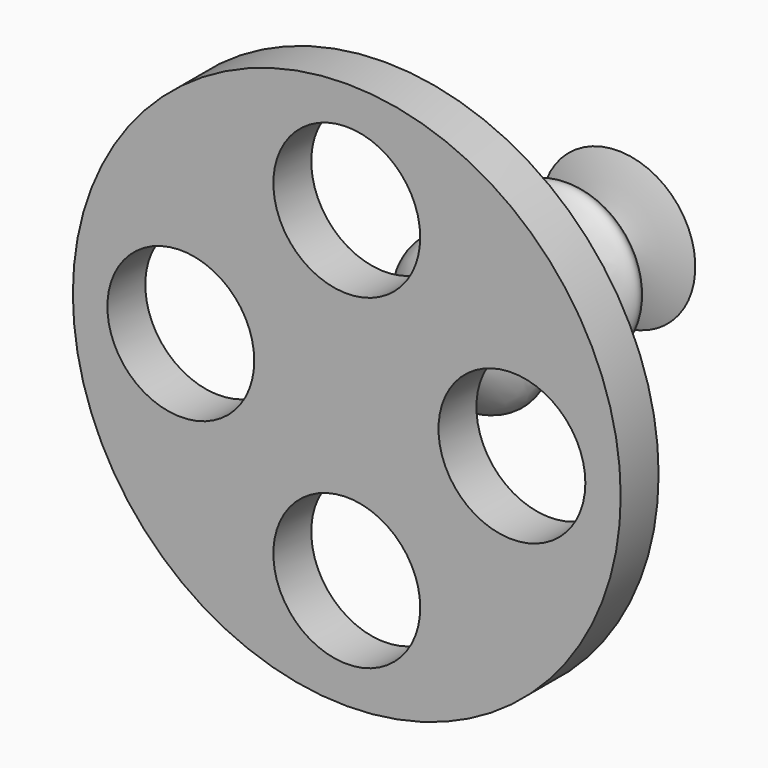
from build123d import *

# Parameters (mm, degrees)
F0_R     = 75.1711608748
F0_R_2   = 20.15
F1_DEPTH = 13


# Not quite as in the source:
# - a feature names something its author has since deleted; it is built from what else it names
# - the program builds the solid bodies; features that only make, move or delete a surface that nothing else refers to are left out


with BuildPart() as f1:
    # F0 (on Front) → F1 (new body)
    with BuildSketch(Plane.XZ):
        Circle(F0_R)
        with Locations((0, -44.8568575084)):
            Circle(F0_R_2, mode=Mode.SUBTRACT)
        with Locations((-45.5452017486, 0)):
            Circle(F0_R_2, mode=Mode.SUBTRACT)
        with Locations((45.3157536685, 0)):
            Circle(F0_R_2, mode=Mode.SUBTRACT)
        with Locations((0, 44.6274131536)):
            Circle(F0_R_2, mode=Mode.SUBTRACT)
    extrude(amount=F1_DEPTH)

    # F2 (on Top) → F3 (revolve)
    with BuildSketch(Plane.XY):
        with BuildLine():
            Line((-21.1639329791, 0), (0, 0))
            Line((0, 0), (0, 80.0915658474))
            Line((0, 80.0915658474), (-21.1639329791, 80.0915658474))
            add(Edge.make_bspline(
                [(-21.1639329791, 0), (-19.2742553322, 4.6189694115), (3.1468380819, 14.4620732239), (-34.8000145769, 30.7354101763), (8.134922476, 47.7855342492), (-36.319607523, 61.0135638885), (9.834598536, 75.0191615104), (-16.6499702233, 77.9874063736), (-21.1639329791, 80.0915658474)],
                knots=[0, 0, 0, 0, 0.1626396624, 0.3304383742, 0.5058929878, 0.6723966985, 0.8424869218, 1, 1, 1, 1], degree=3))
        make_face()
    revolve(axis=Axis((0, 40.0457829237, 0), (0, 1, 0)))


solid = f1.part
